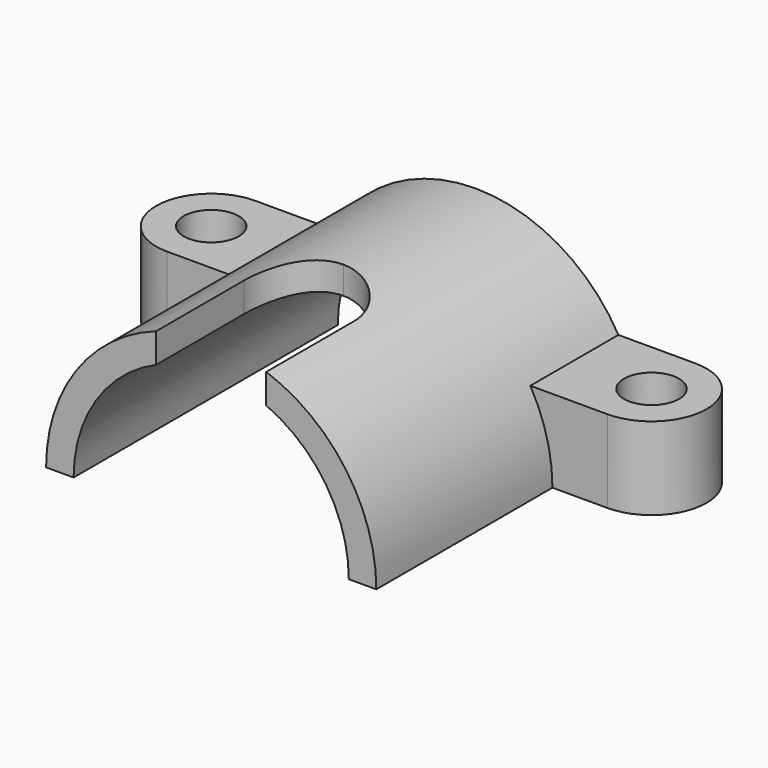
from build123d import *

# Parameters (mm, degrees)
F1_DEPTH = 60
F3_DEPTH = 15
F4_R     = 5
F5_DEPTH = 15
F7_DEPTH = 30.0010001
F8_R     = 25
F9_DEPTH = 60.0010001


# Not quite as in the source:
# - a pattern or mirror of a feature is missing from the dataset's text; its kind, count and spacing are read off the source's solid


with BuildPart() as f1:
    # F0 (on Front) → F1 (new body)
    with BuildSketch(Plane.XZ):
        with BuildLine():
            Line((-30, 0), (30, 0))
            ThreePointArc((30, 0), (0, 30), (-30, 0))
        make_face()
    extrude(amount=-F1_DEPTH)

    # F2 (on Top) → F3 (join)
    with BuildSketch(Plane.XY):
        with BuildLine():
            ThreePointArc((-40, 60), (-50, 50), (-40, 40))
            Line((-40, 40), (40, 40))
            ThreePointArc((40, 40), (50, 50), (40, 60))
            Line((40, 60), (-40, 60))
        make_face()
    extrude(amount=F3_DEPTH)

    # F4 (on Top) → F5 (cut, through all)
    with BuildSketch(Plane.XY):
        with Locations((-40, 50)):
            Circle(F4_R)
    f5 = extrude(amount=F5_DEPTH, mode=Mode.SUBTRACT)

    # F5_copies: F5 across plane
    add(f5.mirror(Plane(origin=(0, 0, 0), x_dir=(0, 0, 1), z_dir=(1, 0, 0))), mode=Mode.SUBTRACT)

    # F6 (on Top) → F7 (cut, through all)
    with BuildSketch(Plane.XY):
        with BuildLine():
            Line((-10, 20), (-10, 0))
            Line((-10, 0), (0, 0))
            Line((0, 0), (0, 30))
            ThreePointArc((0, 30), (-7.0710678119, 27.0710678119), (-10, 20))
        make_face()
        with BuildLine():
            Line((0, 30), (0, 0))
            Line((0, 0), (10, 0))
            Line((10, 0), (10, 20))
            ThreePointArc((10, 20), (7.0710678119, 27.0710678119), (0, 30))
        make_face()
    extrude(amount=F7_DEPTH, mode=Mode.SUBTRACT)

    # F8 (on face) → F9 (cut, through all)
    with BuildSketch(Plane.XZ):
        Circle(F8_R)
    extrude(amount=-F9_DEPTH, mode=Mode.SUBTRACT)


solid = f1.part
